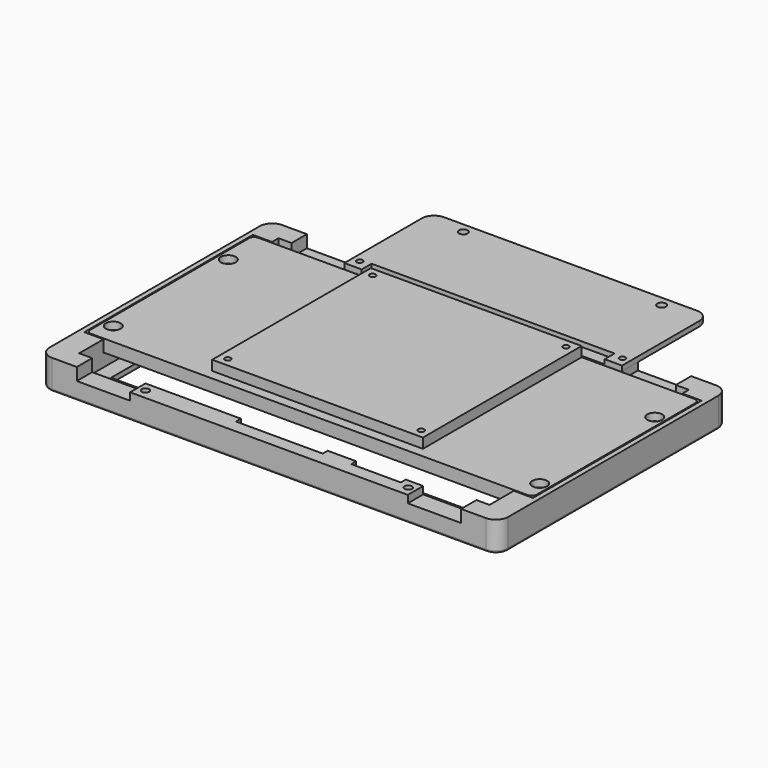
from build123d import *

# Parameters (mm, degrees)
F0_W            = 185
F0_H            = 116
F1_DEPTH        = 12
F2_W            = 20
F2_H            = 2.5
F2_W_2          = 35
F3_DEPTH        = 10
F4_W            = 153
F4_H            = 88
F5_DEPTH        = 25
F6_W            = 181
F6_H            = 85
F7_DEPTH        = 5
F8_W            = 180
F8_H            = 84
F9_DEPTH        = 5
F10_R           = 5
F12_D           = 3
F12_DEPTH       = 20
F12_CBORE_D     = 6
F12_CBORE_DEPTH = 3
F12_TIP         = 0.9012909285
F11_R           = 1.2
F13_DEPTH       = 10
F15_W           = 112
F15_H           = 116
F16_DEPTH       = 2
F18_D           = 3
F18_DEPTH       = 30
F18_CBORE_D     = 6
F18_CBORE_DEPTH = 4
F18_TIP         = 0.9012909285
F19_W           = 21.5
F19_H           = 7.75
F20_DEPTH       = 5
F21_W           = 112
F21_H           = 44
F21_R           = 1.2
F21_R_2         = 1.75
F22_DEPTH       = 2
F23_R           = 5
F24_W           = 85
F24_H           = 80
F25_DEPTH       = 4
F26_R           = 1.2
F27_DEPTH       = 6
F28_R           = 2
F29_W           = 98
F29_H           = 5
F30_DEPTH       = 2
F31_R           = 0.99999


# Not quite as in the source:
# - a fillet or chamfer is up to 0.001 mm smaller than in the source, because OpenCascade refuses the exact size


with BuildPart() as f1:
    # F0 (on Top) → F1 (new body)
    with BuildSketch(Plane.XY):
        Rectangle(F0_W, F0_H)
    extrude(amount=F1_DEPTH)

    # F2 (on face) → F3 (cut)
    with BuildSketch(Plane.XY.offset(12)):
        Polygon((49, -50.25), (82.75, -50.25), (82.75, 50.25), (-82.75, 50.25), (-82.75, -50.25), (-17.5, -50.25), (17.5, -50.25), (29, -50.25), align=None)
        with Locations((39, -51.5)):
            Rectangle(F2_W, F2_H)
        with Locations((0, -51.5)):
            Rectangle(F2_W_2, F2_H)
    extrude(amount=-F3_DEPTH, mode=Mode.SUBTRACT)

    # F4 (on face) → F5 (cut)
    with BuildSketch(Plane(origin=(0, 0, 0), x_dir=(1, 0, 0), z_dir=(0, 0, -1))):
        with Locations((0, -2)):
            Rectangle(F4_W, F4_H)
    extrude(amount=-F5_DEPTH, mode=Mode.SUBTRACT)

    # F6 (on face) → F7 (cut)
    with BuildSketch(Plane.XY.offset(12)):
        with Locations((0, 4.5)):
            Rectangle(F6_W, F6_H)
    extrude(amount=-F7_DEPTH, mode=Mode.SUBTRACT)

    # F10
    f10_edges = [f1.edges().sort_by_distance(p)[0] for p in [
        (-92.5, 58, 6),
        (92.5, 58, 6),
        (92.5, -58, 6),
        (-92.5, -58, 6),
    ]]
    fillet(f10_edges, radius=F10_R)

    # F11 (on face) → F13 (cut)
    with BuildSketch(Plane.XY.offset(12)):
        with Locations((-86, 29)):
            Circle(F11_R)
        with Locations((-86, -29)):
            Circle(F11_R)
        with Locations((86, -29)):
            Circle(F11_R)
        with Locations((86, 29)):
            Circle(F11_R)
    extrude(amount=-F13_DEPTH, mode=Mode.SUBTRACT)

    # F15 (on face) → F16 (cut)
    with BuildSketch(Plane.XY.offset(12)):
        Rectangle(F15_W, F15_H)
    extrude(amount=-F16_DEPTH, mode=Mode.SUBTRACT)

    # F18
    with Locations(Plane(origin=(0, 0, 0), x_dir=(1, 0, 0), z_dir=(0, 0, -1))):
        with Locations((-53, 54), (-53, -54), (53, 54), (53, -54)):
            CounterBoreHole(F18_D / 2, F18_CBORE_D / 2, F18_CBORE_DEPTH, depth=F18_DEPTH)
            with Locations((0, 0, -(F18_DEPTH + F18_TIP / 2))):  # 118° drill point
                Cone(0, F18_D / 2, F18_TIP, mode=Mode.SUBTRACT)

    # F19 (on face) → F20 (cut)
    with BuildSketch(Plane.XY.offset(12)):
        with Locations((-66.75, 54.125)):
            Rectangle(F19_W, F19_H)
        with Locations((-66.75, -54.125)):
            Rectangle(F19_W, F19_H)
        with Locations((66.75, 54.125)):
            Rectangle(F19_W, F19_H)
        with Locations((66.75, -54.125)):
            Rectangle(F19_W, F19_H)
    extrude(amount=-F20_DEPTH, mode=Mode.SUBTRACT)

    # F31 (radius 1 in the source; OpenCascade refuses exactly that, so slightly less here)
    f31_edges = [f1.edges().sort_by_distance(p)[0] for p in [
        (0, -58, 0),
        (-91.035534, -56.535534, 0),
        (91.035534, -56.535534, 0),
        (-92.5, 0, 0),
        (92.5, 0, 0),
        (-91.035534, 56.535534, 0),
        (91.035534, 56.535534, 0),
        (0, 58, 0),
    ]]
    fillet(f31_edges, radius=F31_R)


with BuildPart() as f9:
    # F8 (on face) → F9 (new body)
    with BuildSketch(Plane.XY.offset(7)):
        with Locations((0, 4.5)):
            Rectangle(F8_W, F8_H)
    extrude(amount=F9_DEPTH)

    # F12
    with Locations(Plane.XY.offset(12)):
        with Locations((-86, 29), (-86, -29), (86, 29), (86, -29)):
            CounterBoreHole(F12_D / 2, F12_CBORE_D / 2, F12_CBORE_DEPTH, depth=F12_DEPTH)
            with Locations((0, 0, -(F12_DEPTH + F12_TIP / 2))):  # 118° drill point
                Cone(0, F12_D / 2, F12_TIP, mode=Mode.SUBTRACT)

    # F24 (on face) → F25 (join)
    with BuildSketch(Plane.XY.offset(12)):
        with Locations((0, 6.5)):
            Rectangle(F24_W, F24_H)
    extrude(amount=F25_DEPTH)

    # F26 (on face) → F27 (cut)
    with BuildSketch(Plane.XY.offset(16)):
        with Locations((-39, 43)):
            Circle(F26_R)
        with Locations((39, 43)):
            Circle(F26_R)
        with Locations((-39, -30)):
            Circle(F26_R)
        with Locations((39, -30)):
            Circle(F26_R)
    extrude(amount=-F27_DEPTH, mode=Mode.SUBTRACT)

    # F28
    f28_edges = [f9.edges().sort_by_distance(p)[0] for p in [
        (-90, 46.5, 9.5),
        (-90, -37.5, 9.5),
        (90, -37.5, 9.5),
        (90, 46.5, 9.5),
    ]]
    fillet(f28_edges, radius=F28_R)


with BuildPart() as f22:
    # F21 (on face) → F22 (new body)
    with BuildSketch(Plane.XY.offset(10)):
        with Locations((0, 72)):
            Rectangle(F21_W, F21_H)
        with Locations((-53, 54)):
            Circle(F21_R, mode=Mode.SUBTRACT)
        with Locations((53, 54)):
            Circle(F21_R, mode=Mode.SUBTRACT)
        with Locations((-40, 90)):
            Circle(F21_R_2, mode=Mode.SUBTRACT)
        with Locations((40, 90)):
            Circle(F21_R_2, mode=Mode.SUBTRACT)
    extrude(amount=F22_DEPTH)

    # F23
    f23_edges = [f22.edges().sort_by_distance(p)[0] for p in [
        (-56, 94, 11),
        (56, 94, 11),
    ]]
    fillet(f23_edges, radius=F23_R)

    # F29 (on face) → F30 (cut)
    with BuildSketch(Plane.XY.offset(12)):
        with Locations((0, 52.5)):
            Rectangle(F29_W, F29_H)
    extrude(amount=-F30_DEPTH, mode=Mode.SUBTRACT)


solid = Compound([f1.part, f9.part, f22.part])
